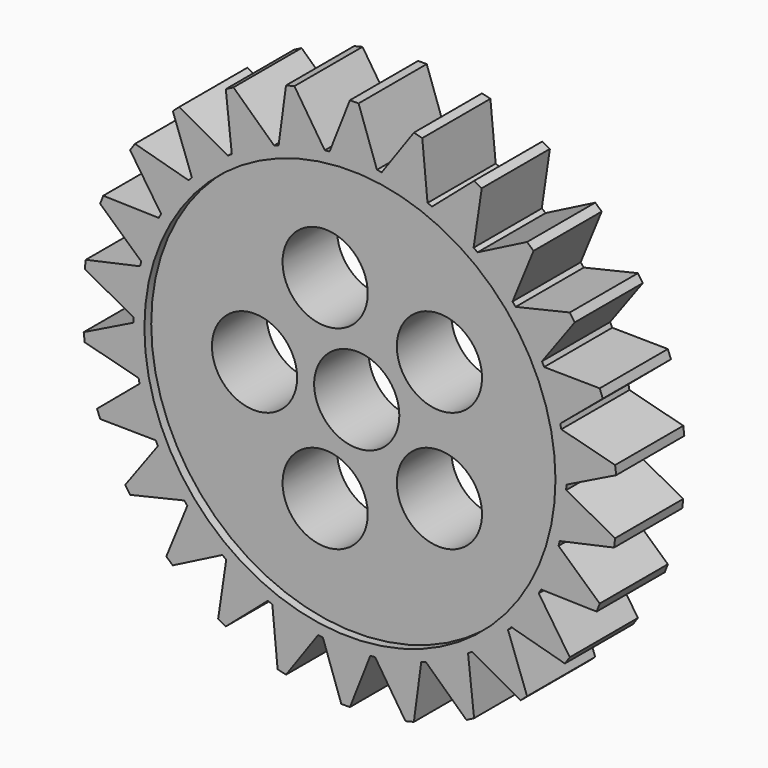
from build123d import *

# Parameters (mm, degrees)
F0_R            = 60.325
F0_R_2          = 12.5
F1_DEPTH        = 10
F2_DEPTH        = 12.5
F3_DEPTH        = 12.5
F3_COPIES_COUNT = 26
F4_R            = 12.5
F5_DEPTH        = 22.501
F5_COPIES_COUNT = 5


# Not quite as in the source:
# - a pattern or mirror of a feature is missing from the dataset's text; its kind, count and spacing are read off the source's solid


with BuildPart() as f1:
    # F0 (on Front) → F1 (new body, symmetric)
    with BuildSketch(Plane.XZ):
        with BuildLine():
            ThreePointArc((-5.9714194874, 63.2186060373), (-42.7379507145, -46.9650675367), (63.5, 0))
            ThreePointArc((63.5, 0), (47.6226622583, 42.0039526644), (7.9304869469, 63.0028362598))
            ThreePointArc((7.9304869469, 63.0028362598), (0.9854569889, 63.4923528822), (-5.9714194874, 63.2186060373))
        make_face()
        Circle(F0_R, mode=Mode.SUBTRACT)
        Circle(F0_R)
        Circle(F0_R_2, mode=Mode.SUBTRACT)
    extrude(amount=F1_DEPTH, both=True)

    # F0 (on Front) → F2 (join, symmetric)
    with BuildSketch(Plane.XZ):
        with BuildLine():
            ThreePointArc((-5.9714194874, 63.2186060373), (-42.7379507145, -46.9650675367), (63.5, 0))
            ThreePointArc((63.5, 0), (47.6226622583, 42.0039526644), (7.9304869469, 63.0028362598))
            ThreePointArc((7.9304869469, 63.0028362598), (0.9854569889, 63.4923528822), (-5.9714194874, 63.2186060373))
        make_face()
        Circle(F0_R, mode=Mode.SUBTRACT)
    extrude(amount=F2_DEPTH, both=True)

    # F0 (on Front) → F3 (join, symmetric)
    with BuildSketch(Plane.XZ):
        with BuildLine():
            ThreePointArc((-5.9714194874, 63.2186060373), (0.9854569889, 63.4923528822), (7.9304869469, 63.0028362598))
            Line((7.9304869469, 63.0028362598), (2.54, 78.4059613943))
            Line((2.54, 78.4059613943), (0, 78.4059613943))
            Line((0, 78.4059613943), (-5.9714194874, 63.2186060373))
        make_face()
    f3 = extrude(amount=F3_DEPTH, both=True)

    # F3_copies: F3 ×26 about axis
    f3_copies_axis = Axis((0, 0, 0), (0, 1, 0))
    for i in range(1, F3_COPIES_COUNT):
        add(f3.rotate(f3_copies_axis, i * 360 / F3_COPIES_COUNT))

    # F4 (on face) → F5 (cut, through all)
    with BuildSketch(Plane.XZ.offset(10)):
        with Locations((-30, 0)):
            Circle(F4_R)
    f5 = extrude(amount=-F5_DEPTH, mode=Mode.SUBTRACT)

    # F5_copies: F5 ×5 about axis
    f5_copies_axis = Axis((0, 0, 0), (0, 1, 0))
    for i in range(1, F5_COPIES_COUNT):
        add(f5.rotate(f5_copies_axis, i * 360 / F5_COPIES_COUNT), mode=Mode.SUBTRACT)


solid = f1.part
